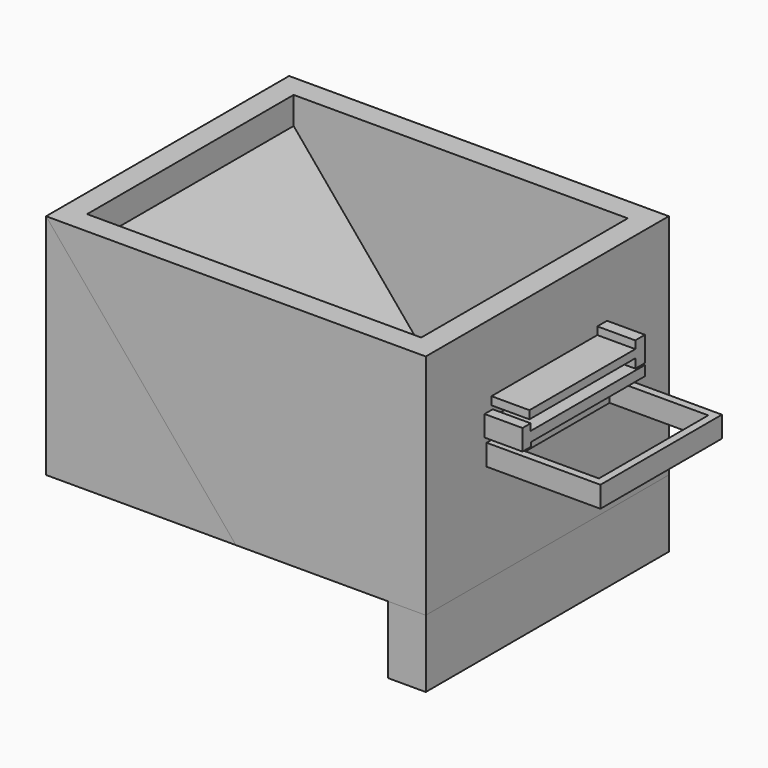
from build123d import *

# Parameters (mm, degrees)
F0_W      = 127
F0_H      = 76.2
F1_DEPTH  = 101.6
F2_W      = 111.76
F2_H      = 86.36
F3_DEPTH  = 66.04
F5_DEPTH  = 25.4
F7_DEPTH  = 22.606
F9_DEPTH  = 101.6
F10_W     = 50.8
F10_H     = 7.0630987705
F11_DEPTH = 38.1
F12_W     = 31.4156402662
F12_H     = 38.1
F13_DEPTH = 50.8
F16_W     = 33.02
F16_H     = 45.72
F16_W_2   = 31.4156402662
F16_H_2   = 38.1
F17_DEPTH = 25.4
F19_DEPTH = 12.7
F21_DEPTH = 12.7


# Not quite as in the source:
# - the program builds the solid bodies; features that only make, move or delete a surface that nothing else refers to are left out


with BuildPart() as f1:
    # F0 (on Front) → F1 (new body)
    with BuildSketch(Plane.XZ):
        with Locations((63.5, 38.1)):
            Rectangle(F0_W, F0_H)
    extrude(amount=-F1_DEPTH)

    # F2 (on face) → F3 (cut)
    with BuildSketch(Plane.XY.offset(76.2)):
        with Locations((63.5, 50.8)):
            Rectangle(F2_W, F2_H)
    extrude(amount=-F3_DEPTH, mode=Mode.SUBTRACT)

    # F4 (on face) → F5 (cut)
    with BuildSketch(Plane(origin=(0, 0, 0), x_dir=(1, 0, 0), z_dir=(0, 0, -1))):
        Polygon((114.3, -12.7), (83.0283915298, -12.7), (83.0283915298, -88.9), (90.3639442819, -88.9), (114.3, -88.9), align=None)
    extrude(amount=-F5_DEPTH, mode=Mode.SUBTRACT)

    # F18 (on face) → F19 (join)
    with BuildSketch(Plane.YZ.offset(127)):
        Polygon((24.5852842927, 49.2701493204), (24.5852842927, 42.3285476863), (28.1094815582, 42.3285476863), (28.1094815582, 43.716866523), (75.7395401597, 43.716866523), (75.7395401597, 47.0274761319), (61.3223686814, 47.0274761319), (28.0026886612, 47.0274761319), (28.0026886612, 49.2701493204), align=None)
    extrude(amount=F19_DEPTH)

    # F20 (on face) → F21 (join)
    with BuildSketch(Plane.YZ.offset(127)):
        Polygon((75.7866054773, 47.5999712944), (75.7866054773, 48.753041774), (75.7866054773, 52.4664781988), (75.7866054773, 55.914670229), (71.7250332236, 55.914670229), (71.7250332236, 53.3474907279), (27.4760443717, 53.3474907279), (27.4760443717, 50.6468489766), (71.7250332236, 50.6468489766), (71.7250332236, 47.5999712944), align=None)
    extrude(amount=F21_DEPTH)


with BuildPart() as f7:
    # F6 (on face) → F7 (new body)
    with BuildSketch(Plane(origin=(0, 0, 0), x_dir=(1, 0, 0), z_dir=(0, 0, -1))):
        Polygon((114.3, 0), (114.3, -12.7), (114.3, -88.9), (114.3, -101.6), (127, -101.6), (127, 0), align=None)
    extrude(amount=F7_DEPTH)


with BuildPart() as f9:
    # F8 (on face) → F9 (new body)
    with BuildSketch(Plane.XZ):
        Polygon((63.5, 0), (0, 76.2), (0, 0), align=None)
    extrude(amount=-F9_DEPTH)


with BuildPart() as f11:
    # F10 (on face) → F11 (new body)
    with BuildSketch(Plane.YZ.offset(127)):
        with Locations((50.8, 36.9570013136)):
            Rectangle(F10_W, F10_H)
    extrude(amount=F11_DEPTH)

    # F12 (on face) → F13 (cut)
    with BuildSketch(Plane.XY.offset(40.4885506988)):
        with Locations((145.3281798669, 50.8)):
            Rectangle(F12_W, F12_H)
    extrude(amount=-F13_DEPTH, mode=Mode.SUBTRACT)

    # F16 (on face) → F17 (cut)
    with BuildSketch(Plane.XY.offset(40.4885506988)):
        with Locations((146.05, 50.8)):
            Rectangle(F16_W, F16_H)
        with Locations((145.3281798669, 50.8)):
            Rectangle(F16_W_2, F16_H_2, mode=Mode.SUBTRACT)
    extrude(amount=-F17_DEPTH, mode=Mode.SUBTRACT)


solid = Compound([f1.part, f7.part, f9.part, f11.part])
